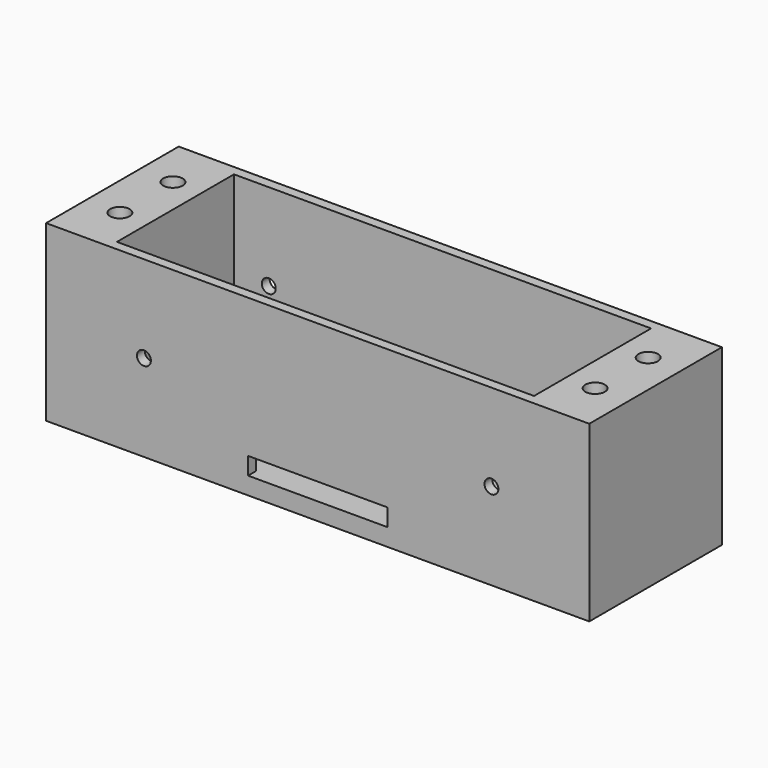
from build123d import *

# Parameters (mm, degrees)
F0_W     = 5
F0_H     = 47.625
F0_W_2   = 146.05
F0_R     = 3.24
F1_DEPTH = 50
F2_W     = 119.824
F2_H     = 42.025
F3_DEPTH = 45
F4_D     = 5.6
F4_DEPTH = 20
F4_TIP   = 1.6824097333
F5_W     = 40
F5_H     = 5
F6_DEPTH = 47.626
F7_D     = 4


# Not quite as in the source:
# - ends of sketch curves that miss each other by under 0.0002 mm in the source are joined


with BuildPart() as f1:
    # F0 (on Top) → F1 (new body)
    with BuildSketch(Plane.XY):
        with Locations((-75.525, 0)):
            Rectangle(F0_W, F0_H)
        Rectangle(F0_W_2, F0_H)
        with Locations((-68.262, -9.5245)):
            Circle(F0_R, mode=Mode.SUBTRACT)
        with Locations((68.262, -9.5245)):
            Circle(F0_R, mode=Mode.SUBTRACT)
        with Locations((-68.262, 9.5245)):
            Circle(F0_R, mode=Mode.SUBTRACT)
        with BuildLine():
            Line((72.225, -15.859485), (72.225, -23.0125))
            Line((72.225, -23.0125), (-72.225, -23.0125))
            Line((-72.225, -23.0125), (-72.225, -15.874133))
            Line((-72.225, -15.874133), (-68.193705, -15.874133))
            ThreePointArc((-68.193705, -15.874133), (-61.912367271, -9.4562050029), (-68.3302949971, -3.174867271))
            Line((-68.3302949971, -3.174867271), (-72.225, -3.174867))
            Line((-72.225, -3.174867), (-72.225, 3.1745))
            Line((-72.225, 3.1745), (-68.262, 3.1745))
            ThreePointArc((-68.262, 3.1745), (-61.912, 9.5245), (-68.262, 15.8745))
            Line((-68.262, 15.8745), (-72.225, 15.8745))
            Line((-72.225, 15.8745), (-72.225, 23.0125))
            Line((-72.225, 23.0125), (72.225, 23.0125))
            Line((72.225, 23.0125), (72.225, 15.8745))
            Line((72.225, 15.8745), (68.262, 15.8745))
            ThreePointArc((68.262, 15.8745), (61.912, 9.5245), (68.262, 3.1745))
            Line((68.262, 3.1745), (72.225, 3.1745))
            Line((72.225, 3.1745), (72.225, -3.189515))
            Line((72.225, -3.189515), (67.825573, -3.189515))
            ThreePointArc((67.825573, -3.189515), (61.9270152731, -9.9609269812), (68.6984269812, -15.8594847269))
            Line((68.6984269812, -15.8594847269), (72.225, -15.859485))
        make_face(mode=Mode.SUBTRACT)
        with Locations((68.262, 9.5245)):
            Circle(F0_R, mode=Mode.SUBTRACT)
        with Locations((75.525, 0)):
            Rectangle(F0_W, F0_H)
        with Locations((-68.262, 9.5245)):
            Circle(F0_R)
        with Locations((-68.262, -9.5245)):
            Circle(F0_R)
        with BuildLine():
            Line((-72.225, -23.0125), (72.225, -23.0125))
            Line((72.225, -23.0125), (72.225, -15.859485))
            Line((72.225, -15.859485), (68.698427, -15.859485))
            ThreePointArc((68.698427, -15.859485), (61.9270152731, -9.9609269812), (67.8255730188, -3.1895152731))
            Line((67.8255730188, -3.1895152731), (72.225, -3.189515))
            Line((72.225, -3.189515), (72.225, 3.1745))
            Line((72.225, 3.1745), (68.262, 3.1745))
            ThreePointArc((68.262, 3.1745), (61.912, 9.5245), (68.262, 15.8745))
            Line((68.262, 15.8745), (72.225, 15.8745))
            Line((72.225, 15.8745), (72.225, 23.0125))
            Line((72.225, 23.0125), (-72.225, 23.0125))
            Line((-72.225, 23.0125), (-72.225, 15.8745))
            Line((-72.225, 15.8745), (-68.262, 15.8745))
            ThreePointArc((-68.262, 15.8745), (-61.912, 9.5245), (-68.262, 3.1745))
            Line((-68.262, 3.1745), (-72.225, 3.1745))
            Line((-72.225, 3.1745), (-72.225, -3.174867))
            Line((-72.225, -3.174867), (-68.330295, -3.174867))
            ThreePointArc((-68.330295, -3.174867), (-61.912367271, -9.4562050029), (-68.1937050029, -15.874132729))
            Line((-68.1937050029, -15.874132729), (-72.225, -15.874133))
            Line((-72.225, -15.874133), (-72.225, -23.0125))
        make_face()
        with Locations((68.262, 9.5245)):
            Circle(F0_R)
        with Locations((68.262, -9.5245)):
            Circle(F0_R)
    extrude(amount=-F1_DEPTH)

    # F2 (on face) → F3 (cut)
    with BuildSketch(Plane.XY):
        Rectangle(F2_W, F2_H)
    extrude(amount=-F3_DEPTH, mode=Mode.SUBTRACT)

    # F4
    with Locations(Plane.XY):
        with Locations((-68.262, 9.5245), (-68.262, -9.5245), (68.262, 9.5245), (68.262, -9.5245)):
            Hole(F4_D / 2, depth=F4_DEPTH)
            with Locations((0, 0, -(F4_DEPTH + F4_TIP / 2))):  # 118° drill point
                Cone(0, F4_D / 2, F4_TIP, mode=Mode.SUBTRACT)

    # F5 (on face) → F6 (cut, through all)
    with BuildSketch(Plane.XZ.offset(23.8125)):
        with Locations((0, -42.5)):
            Rectangle(F5_W, F5_H)
    extrude(amount=-F6_DEPTH, mode=Mode.SUBTRACT)

    # F7 (through all)
    with Locations(Plane.XZ.offset(23.8125)):
        with Locations((-49.912, -25), (49.912, -25)):
            Hole(F7_D / 2)


solid = f1.part
